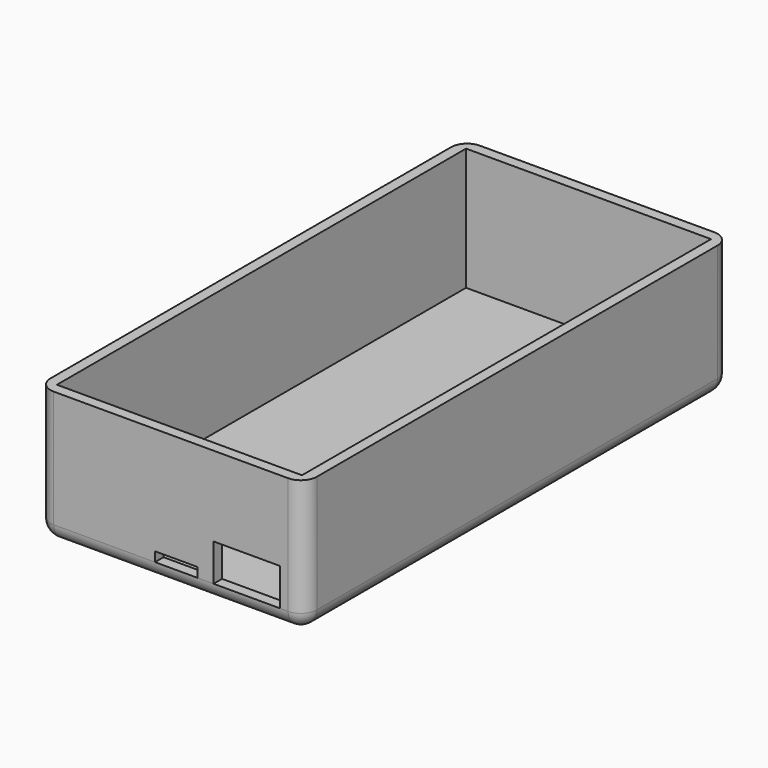
from build123d import *

# Parameters (mm, degrees)
F0_W     = 50
F0_H     = 100
F1_DEPTH = 25
F2_T     = -2
F3_W     = 12.5
F3_H     = 7
F3_W_2   = 8
F3_H_2   = 1.8
F4_DEPTH = 2
F5_R     = 3
F6_R     = 2.99999


# Not quite as in the source:
# - a fillet or chamfer is up to 0.001 mm smaller than in the source, because OpenCascade refuses the exact size


with BuildPart() as f1:
    # F0 (on Top) → F1 (new body)
    with BuildSketch(Plane.XY):
        Rectangle(F0_W, F0_H)
    extrude(amount=F1_DEPTH)

    # F2
    f2_openings = [f1.faces().sort_by_distance(p)[0] for p in [
        (0, 0, 25),
    ]]
    offset(amount=F2_T, openings=f2_openings)

    # F3 (on face) → F4 (cut)
    with BuildSketch(Plane.XZ.offset(50)):
        with Locations((14.25, 6.5)):
            Rectangle(F3_W, F3_H)
        with Locations((1, 3.9)):
            Rectangle(F3_W_2, F3_H_2)
    extrude(amount=-F4_DEPTH, mode=Mode.SUBTRACT)

    # F5
    f5_edges = [f1.edges().sort_by_distance(p)[0] for p in [
        (25, -50, 12.5),
    ]]
    fillet(f5_edges, radius=F5_R)

    # F6 (radius 3 in the source; OpenCascade refuses exactly that, so slightly less here)
    f6_edges = [f1.edges().sort_by_distance(p)[0] for p in [
        (25, 50, 12.5),
        (-25, 50, 12.5),
        (-25, -50, 12.5),
        (-25, 0, 0),
        (-1.5, -50, 0),
        (0, 50, 0),
    ]]
    fillet(f6_edges, radius=F6_R)


solid = f1.part
